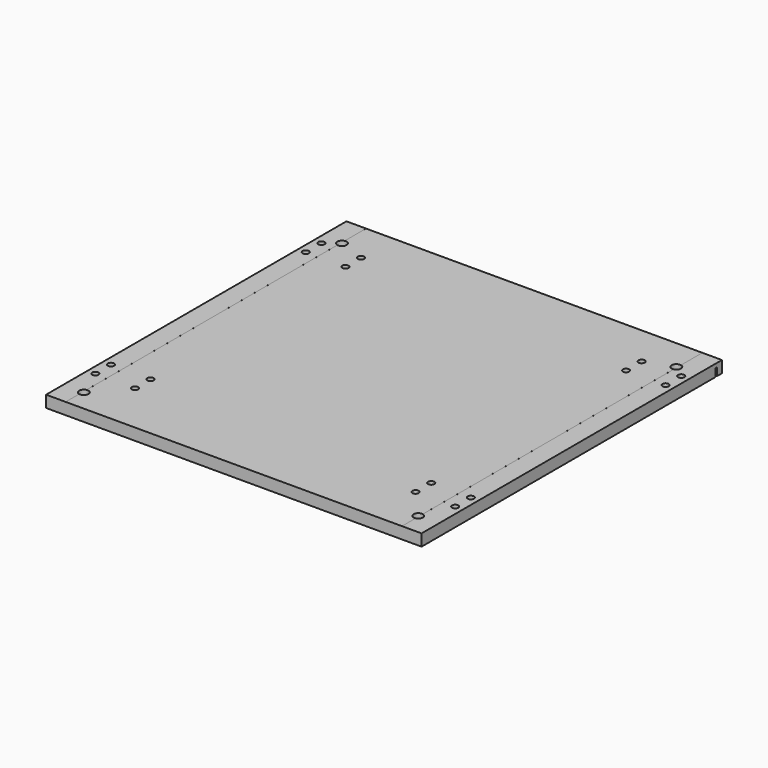
from build123d import *

# Parameters (mm, degrees)
F0_W     = 609.6
F0_H     = 609.6
F0_R     = 7.540625
F0_R_2   = 5.159375
F1_DEPTH = 19.05
F2_DEPTH = 12.7
F3_W     = 609.6
F3_H     = 3.175
F4_DEPTH = 12.7
F5_W     = 25.4
F5_H     = 0.0254
F5_W_2   = 50
F6_DEPTH = 0.254
F8_DEPTH = 2.54


# Not quite as in the source:
# - a pattern or mirror of a feature is missing from the dataset's text; its kind, count and spacing are read off the source's solid
# - a feature names something its author has since deleted; it is built from what else it names


with BuildPart() as f1:
    # F0 (on Top) → F1 (new body)
    with BuildSketch(Plane.XY):
        Rectangle(F0_W, F0_H)
        with Locations((-271.4625, -269.875)):
            Circle(F0_R, mode=Mode.SUBTRACT)
        with Locations((-292.1, -220.6625)):
            Circle(F0_R_2, mode=Mode.SUBTRACT)
        with Locations((-292.1, -188.9125)):
            Circle(F0_R_2, mode=Mode.SUBTRACT)
        with Locations((-227.80625, -220.6625)):
            Circle(F0_R_2, mode=Mode.SUBTRACT)
        with Locations((-227.80625, -188.9125)):
            Circle(F0_R_2, mode=Mode.SUBTRACT)
        with Locations((-292.1, 206.375)):
            Circle(F0_R_2, mode=Mode.SUBTRACT)
        with Locations((-227.80625, 206.375)):
            Circle(F0_R_2, mode=Mode.SUBTRACT)
        with Locations((-292.1, 238.125)):
            Circle(F0_R_2, mode=Mode.SUBTRACT)
        with Locations((-271.4625, 254)):
            Circle(F0_R, mode=Mode.SUBTRACT)
        with Locations((-227.80625, 238.125)):
            Circle(F0_R_2, mode=Mode.SUBTRACT)
        with Locations((-227.80625, 206.375)):
            Circle(F0_R_2)
        with Locations((-227.80625, 238.125)):
            Circle(F0_R_2)
        with Locations((-227.80625, -188.9125)):
            Circle(F0_R_2)
        with Locations((-227.80625, -220.6625)):
            Circle(F0_R_2)
        with Locations((-271.4625, -269.875)):
            Circle(F0_R)
        with Locations((-271.4625, 254)):
            Circle(F0_R)
        with Locations((-292.1, 238.125)):
            Circle(F0_R_2)
        with Locations((-292.1, 206.375)):
            Circle(F0_R_2)
        with Locations((-292.1, -220.6625)):
            Circle(F0_R_2)
        with Locations((-292.1, -188.9125)):
            Circle(F0_R_2)
    extrude(amount=-F1_DEPTH)

    # F0 (on Top) → F2 (cut)
    with BuildSketch(Plane.XY):
        with Locations((-271.4625, -269.875)):
            Circle(F0_R)
        with Locations((-292.1, -220.6625)):
            Circle(F0_R_2)
        with Locations((-227.80625, -220.6625)):
            Circle(F0_R_2)
        with Locations((-227.80625, -188.9125)):
            Circle(F0_R_2)
        with Locations((-292.1, -188.9125)):
            Circle(F0_R_2)
        with Locations((-292.1, 206.375)):
            Circle(F0_R_2)
        with Locations((-227.80625, 206.375)):
            Circle(F0_R_2)
        with Locations((-227.80625, 238.125)):
            Circle(F0_R_2)
        with Locations((-292.1, 238.125)):
            Circle(F0_R_2)
        with Locations((-271.4625, 254)):
            Circle(F0_R)
    f2 = extrude(amount=-F2_DEPTH, mode=Mode.SUBTRACT)

    # F2_copies: F2 across plane
    add(f2.mirror(Plane(origin=(0, 0, 0), x_dir=(0, 0, 1), z_dir=(1, 0, 0))), mode=Mode.SUBTRACT)

    # F3 (on face) → F4 (cut)
    with BuildSketch(Plane(origin=(0, 0, -19.05), x_dir=(1, 0, 0), z_dir=(0, 0, -1))):
        with Locations((0, -293.6875)):
            Rectangle(F3_W, F3_H)
    extrude(amount=-F4_DEPTH, mode=Mode.SUBTRACT)

    # F5 (on face) → F6 (cut)
    with BuildSketch(Plane(origin=(0, 0, -19.05), x_dir=(1, 0, 0), z_dir=(0, 0, -1))):
        with Locations((-156.0546457767, -265.0721735465)):
            Rectangle(F5_W, F5_H)
        with Locations((-145.1898425817, -234.882380328)):
            Rectangle(F5_W_2, F5_H)
    extrude(amount=-F6_DEPTH, mode=Mode.SUBTRACT)

    # F7 (on face) → F8 (cut)
    with BuildSketch(Plane.XY):
        with BuildLine():
            Line((273.05, 304.8), (273.0246, 304.8))
            Line((273.0246, 304.8), (273.0246, 261.3770501544))
            ThreePointArc((273.0246, 261.3770501544), (273.0373023354, 261.3743489879), (273.05, 261.3716259496))
            Line((273.05, 261.3716259496), (273.05, 304.8))
        make_face()
        with BuildLine():
            ThreePointArc((273.05, 261.3716259496), (273.0373023354, 261.3743489879), (273.0246, 261.3770501544))
            Line((273.0246, 261.3770501544), (273.0246, 246.6229498456))
            ThreePointArc((273.0246, 246.6229498456), (273.0373023354, 246.6256510121), (273.05, 246.6283740504))
            Line((273.05, 246.6283740504), (273.05, 261.3716259496))
        make_face()
        with BuildLine():
            ThreePointArc((273.05, 246.6283740504), (273.0373023354, 246.6256510121), (273.0246, 246.6229498456))
            Line((273.0246, 246.6229498456), (273.0246, -262.4979498456))
            ThreePointArc((273.0246, -262.4979498456), (273.0373023354, -262.5006510121), (273.05, -262.5033740504))
            Line((273.05, -262.5033740504), (273.05, 246.6283740504))
        make_face()
        with BuildLine():
            ThreePointArc((273.05, -262.5033740504), (273.0373023354, -262.5006510121), (273.0246, -262.4979498456))
            Line((273.0246, -262.4979498456), (273.0246, -277.2520501544))
            ThreePointArc((273.0246, -277.2520501544), (273.0373023354, -277.2493489879), (273.05, -277.2466259496))
            Line((273.05, -277.2466259496), (273.05, -262.5033740504))
        make_face()
        with BuildLine():
            Line((273.0246, -277.2520501544), (273.0246, -304.8))
            Line((273.0246, -304.8), (273.05, -304.8))
            Line((273.05, -304.8), (273.05, -277.2466259496))
            ThreePointArc((273.05, -277.2466259496), (273.0373023354, -277.2493489879), (273.0246, -277.2520501544))
        make_face()
        with BuildLine():
            Line((-273.0246, 304.8), (-273.05, 304.8))
            Line((-273.05, 304.8), (-273.05, 261.3716259496))
            ThreePointArc((-273.05, 261.3716259496), (-273.0373023354, 261.3743489879), (-273.0246, 261.3770501544))
            Line((-273.0246, 261.3770501544), (-273.0246, 304.8))
        make_face()
        with BuildLine():
            ThreePointArc((-273.0246, 261.3770501544), (-273.0373023354, 261.3743489879), (-273.05, 261.3716259496))
            Line((-273.05, 261.3716259496), (-273.05, 246.6283740504))
            ThreePointArc((-273.05, 246.6283740504), (-273.0373023354, 246.6256510121), (-273.0246, 246.6229498456))
            Line((-273.0246, 246.6229498456), (-273.0246, 261.3770501544))
        make_face()
        with BuildLine():
            ThreePointArc((-273.0246, -262.4979498456), (-273.0373023354, -262.5006510121), (-273.05, -262.5033740504))
            Line((-273.05, -262.5033740504), (-273.05, -277.2466259496))
            ThreePointArc((-273.05, -277.2466259496), (-273.0373023354, -277.2493489879), (-273.0246, -277.2520501544))
            Line((-273.0246, -277.2520501544), (-273.0246, -262.4979498456))
        make_face()
        with BuildLine():
            Line((-273.05, -277.2466259496), (-273.05, -304.8))
            Line((-273.05, -304.8), (-273.0246, -304.8))
            Line((-273.0246, -304.8), (-273.0246, -277.2520501544))
            ThreePointArc((-273.0246, -277.2520501544), (-273.0373023354, -277.2493489879), (-273.05, -277.2466259496))
        make_face()
        with BuildLine():
            ThreePointArc((-273.0246, 246.6229498456), (-273.0373023354, 246.6256510121), (-273.05, 246.6283740504))
            Line((-273.05, 246.6283740504), (-273.05, -262.5033740504))
            ThreePointArc((-273.05, -262.5033740504), (-273.0373023354, -262.5006510121), (-273.0246, -262.4979498456))
            Line((-273.0246, -262.4979498456), (-273.0246, 246.6229498456))
        make_face()
    extrude(amount=-F8_DEPTH, mode=Mode.SUBTRACT)


solid = f1.part
